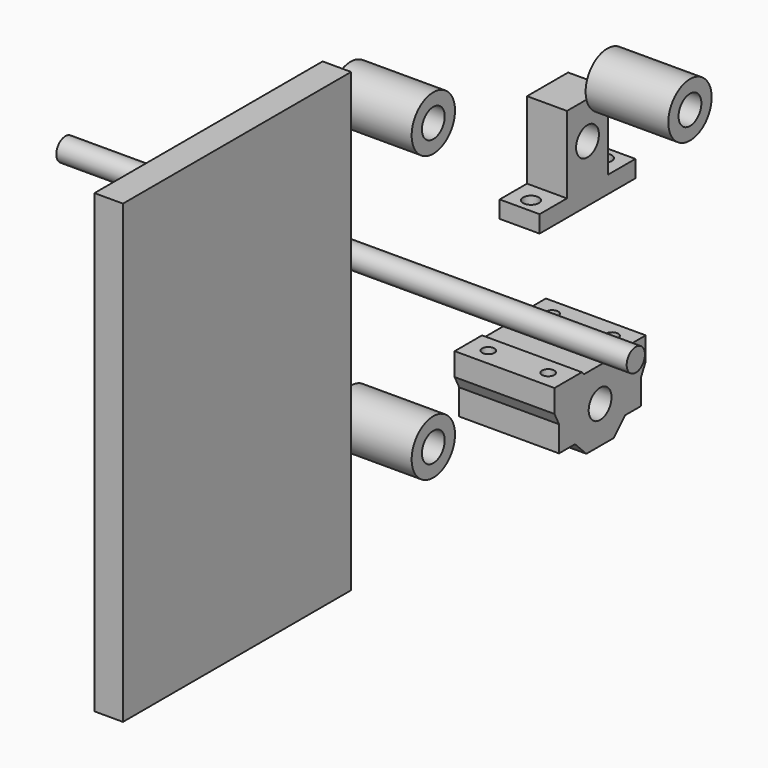
from build123d import *

# Parameters (mm, degrees)
F0_R      = 9.5
F0_R_2    = 5
F1_DEPTH  = 29
F0_R_3    = 4
F2_DEPTH  = 100
F3_DEPTH  = 29
F0_W      = 100
F0_H      = 160
F4_DEPTH  = 10
F5_DEPTH  = 14
F6_R      = 2.75
F7_DEPTH  = 85.8391930217
F8_DEPTH  = 35
F9_R      = 2.15
F10_DEPTH = 133.9749894867


with BuildPart() as f1:
    # F0 (on Right) → F1 (new body)
    with BuildSketch(Plane.YZ):
        with Locations((0, 50)):
            Circle(F0_R)
        with Locations((0, 50)):
            Circle(F0_R_2, mode=Mode.SUBTRACT)
    extrude(amount=F1_DEPTH)


with BuildPart() as f2:
    # F0 (on Right) → F2 (new body, symmetric)
    with BuildSketch(Plane.YZ):
        Circle(F0_R_3)
    extrude(amount=F2_DEPTH, both=True)


with BuildPart() as f3:
    # F0 (on Right) → F3 (new body)
    with BuildSketch(Plane.YZ):
        with Locations((0, -50)):
            Circle(F0_R)
        with Locations((0, -50)):
            Circle(F0_R_2, mode=Mode.SUBTRACT)
    extrude(amount=F3_DEPTH)


with BuildPart() as f4:
    # F0 (on Right) → F4 (new body)
    with BuildSketch(Plane.YZ):
        with Locations((-62.2850701213, -15.426402986)):
            Rectangle(F0_W, F0_H)
    extrude(amount=F4_DEPTH)


with BuildPart() as f5:
    # F0 (on Right) → F5 (new body)
    with BuildSketch(Plane.YZ):
        Polygon((95.3264095187, 17.4117900357), (77.3264095187, 17.4117900357), (77.3264095187, -9.5882099643), (65.3264095187, -9.5882099643), (65.3264095187, -15.5882099643), (107.3264095187, -15.5882099643), (107.3264095187, -9.5882099643), (95.3264095187, -9.5882099643), align=None)
        with Locations((86.3264095187, 4.4117900357)):
            Circle(F0_R_2, mode=Mode.SUBTRACT)
    extrude(amount=F5_DEPTH)

    # F6 (on face) → F7 (cut, through all)
    with BuildSketch(Plane.XY.offset(-9.5882099643)):
        with Locations((7, 102.3264095187)):
            Circle(F6_R)
        with Locations((7, 70.3264095187)):
            Circle(F6_R)
    extrude(amount=-F7_DEPTH, mode=Mode.SUBTRACT)


with BuildPart() as f8:
    # F0 (on Right) → F8 (new body)
    with BuildSketch(Plane.YZ):
        Polygon((57.5972360969, -48.4003924727), (45.5972360969, -48.4003924727), (45.5972360969, -56.4003924727), (47.5972360969, -60.4003924727), (47.5972360969, -69.4003924727), (54.5972360969, -69.4003924727), (59.5972360969, -74.4003924727), (71.5972360969, -74.4003924727), (76.5972360969, -69.4003924727), (83.5972360969, -69.4003924727), (83.5972360969, -60.4003924727), (85.5972360969, -56.4003924727), (85.5972360969, -48.4003924727), (73.5972360969, -48.4003924727), (72.5972360969, -49.4003924727), (58.5972360969, -49.4003924727), align=None)
        with Locations((65.5972360969, -61.4003924727)):
            Circle(F0_R_2, mode=Mode.SUBTRACT)
    extrude(amount=F8_DEPTH)

    # F9 (on face) → F10 (cut, through all)
    with BuildSketch(Plane(origin=(0, 0, -69.4003924727), x_dir=(1, 0, 0), z_dir=(0, 0, -1))):
        with Locations((28, -51.5972360969)):
            Circle(F9_R)
        with Locations((7, -51.5972360969)):
            Circle(F9_R)
        with Locations((28, -79.5972360969)):
            Circle(F9_R)
        with Locations((7, -79.5972360969)):
            Circle(F9_R)
    extrude(amount=-F10_DEPTH, mode=Mode.SUBTRACT)


with BuildPart() as f11_1:
    # F11: copy of F1
    add(f1.part.moved(Location((50, 50, 0))))


solid = Compound([f1.part, f2.part, f3.part, f4.part, f5.part, f8.part, f11_1.part])
